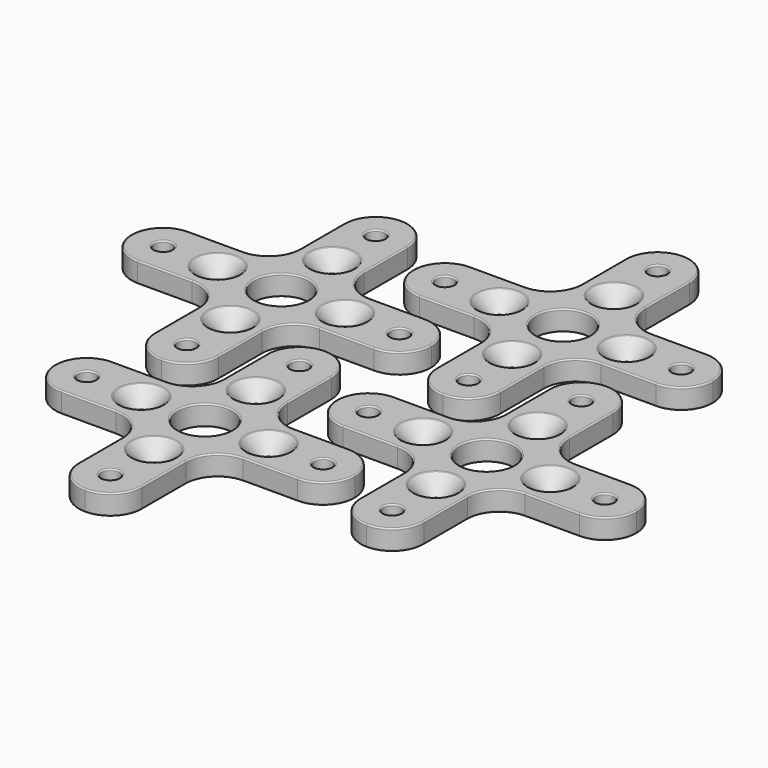
from build123d import *

# Parameters (mm, degrees)
F0_R     = 1
F0_R_2   = 0.8
F0_R_3   = 3
F1_DEPTH = 2.25
F2_R     = 3.49999
F3_SIZE  = 1.7
F4_R     = 0.15


# Not quite as in the source:
# - a fillet or chamfer is up to 0.001 mm smaller than in the source, because OpenCascade refuses the exact size


with BuildPart() as f1:
    # F0 (on Top) → F1 (new body)
    with BuildSketch(Plane.XY):
        Polygon((-53.7742620409, -53.6278340276), (-46.7742620409, -53.6278340276), (-46.7742620409, -40.6278340276), (-33.7742620409, -40.6278340276), (-33.7742620409, -33.6278340276), (-46.7742620409, -33.6278340276), (-46.7742620409, -20.6278340276), (-53.7742620409, -20.6278340276), (-53.7742620409, -33.6278340276), (-66.7742620409, -33.6278340276), (-66.7742620409, -40.6278340276), (-53.7742620409, -40.6278340276), align=None)
        with Locations((-50.2742620409, -50.1278340276)):
            Circle(F0_R, mode=Mode.SUBTRACT)
        with Locations((-50.2742620409, -44.1278340276)):
            Circle(F0_R_2, mode=Mode.SUBTRACT)
        with Locations((-63.2742620409, -37.1278340276)):
            Circle(F0_R, mode=Mode.SUBTRACT)
        with Locations((-57.2742620409, -37.1278340276)):
            Circle(F0_R_2, mode=Mode.SUBTRACT)
        with Locations((-50.2742620409, -37.1278340276)):
            Circle(F0_R_3, mode=Mode.SUBTRACT)
        with Locations((-50.2742620409, -30.1278340276)):
            Circle(F0_R_2, mode=Mode.SUBTRACT)
        with Locations((-50.2742620409, -24.1278340276)):
            Circle(F0_R, mode=Mode.SUBTRACT)
        with Locations((-43.2742620409, -37.1278340276)):
            Circle(F0_R_2, mode=Mode.SUBTRACT)
        with Locations((-37.2742620409, -37.1278340276)):
            Circle(F0_R, mode=Mode.SUBTRACT)
    extrude(amount=F1_DEPTH)

    # F2 (radius 3.5 in the source; OpenCascade refuses exactly that, so slightly less here)
    f2_edges = [f1.edges().sort_by_distance(p)[0] for p in [
        (-53.774262, -20.627834, 1.125),
        (-46.774262, -20.627834, 1.125),
        (-33.774262, -33.627834, 1.125),
        (-33.774262, -40.627834, 1.125),
        (-46.774262, -53.627834, 1.125),
        (-53.774262, -53.627834, 1.125),
        (-66.774262, -40.627834, 1.125),
        (-66.774262, -33.627834, 1.125),
        (-53.774262, -40.627834, 1.125),
        (-46.774262, -40.627834, 1.125),
        (-46.774262, -33.627834, 1.125),
        (-53.774262, -33.627834, 1.125),
    ]]
    fillet(f2_edges, radius=F2_R)

    # F3
    f3_edges = [f1.edges().sort_by_distance(p)[0] for p in [
        (-51.074262, -30.127834, 2.25),
        (-44.074262, -37.127834, 2.25),
        (-51.074262, -44.127834, 2.25),
        (-58.074262, -37.127834, 2.25),
    ]]
    chamfer(f3_edges, length=F3_SIZE)

    # F4
    f4_edges = [f1.edges().sort_by_distance(p)[0] for p in [
        (-52.774262, -30.127834, 2.25),
        (-60.274262, -40.627834, 2.25),
        (-65.749139, -39.602711, 2.25),
        (-54.799385, -41.652957, 2.25),
        (-66.774262, -37.127834, 2.25),
        (-53.774262, -47.127834, 2.25),
        (-65.749139, -34.652957, 2.25),
        (-52.749139, -52.602711, 2.25),
        (-60.274262, -33.627834, 2.25),
        (-50.274262, -53.627834, 2.25),
        (-54.799385, -32.602711, 2.25),
        (-47.799385, -52.602711, 2.25),
        (-53.774262, -27.127834, 2.25),
        (-46.774262, -47.127834, 2.25),
        (-52.749139, -21.652957, 2.25),
        (-45.749139, -41.652957, 2.25),
        (-50.274262, -20.627834, 2.25),
        (-40.274262, -40.627834, 2.25),
        (-47.799385, -21.652957, 2.25),
        (-34.799385, -39.602711, 2.25),
        (-46.774262, -27.127834, 2.25),
        (-33.774262, -37.127834, 2.25),
        (-45.749139, -32.602711, 2.25),
        (-34.799385, -34.652957, 2.25),
        (-40.274262, -33.627834, 2.25),
        (-51.274262, -50.127834, 2.25),
        (-64.274262, -37.127834, 2.25),
        (-53.274262, -37.127834, 2.25),
        (-51.274262, -24.127834, 2.25),
        (-38.274262, -37.127834, 2.25),
        (-45.774262, -37.127834, 2.25),
        (-52.774262, -44.127834, 2.25),
        (-59.774262, -37.127834, 2.25),
        (-60.274262, -40.627834, 0),
        (-65.749139, -39.602711, 0),
        (-54.799385, -41.652957, 0),
        (-66.774262, -37.127834, 0),
        (-53.774262, -47.127834, 0),
        (-65.749139, -34.652957, 0),
        (-52.749139, -52.602711, 0),
        (-60.274262, -33.627834, 0),
        (-50.274262, -53.627834, 0),
        (-54.799385, -32.602711, 0),
        (-47.799385, -52.602711, 0),
        (-53.774262, -27.127834, 0),
        (-46.774262, -47.127834, 0),
        (-52.749139, -21.652957, 0),
        (-45.749139, -41.652957, 0),
        (-50.274262, -20.627834, 0),
        (-40.274262, -40.627834, 0),
        (-47.799385, -21.652957, 0),
        (-34.799385, -39.602711, 0),
        (-46.774262, -27.127834, 0),
        (-33.774262, -37.127834, 0),
        (-45.749139, -32.602711, 0),
        (-34.799385, -34.652957, 0),
        (-40.274262, -33.627834, 0),
        (-51.274262, -50.127834, 0),
        (-51.074262, -44.127834, 0),
        (-64.274262, -37.127834, 0),
        (-58.074262, -37.127834, 0),
        (-53.274262, -37.127834, 0),
        (-51.074262, -30.127834, 0),
        (-51.274262, -24.127834, 0),
        (-44.074262, -37.127834, 0),
        (-38.274262, -37.127834, 0),
    ]]
    fillet(f4_edges, radius=F4_R)


with BuildPart() as f5_1:
    # F5: copy of F1
    add(f1.part.moved(Location((23, 10, 0))))


with BuildPart() as f6_1:
    # F6: copy of F5_1
    add(f5_1.part.moved(Location((10, -23, 0))))


with BuildPart() as f7_1:
    # F7: copy of F6_1
    add(f6_1.part.moved(Location((-23, -10, 0))))


solid = Compound([f1.part, f5_1.part, f6_1.part, f7_1.part])
